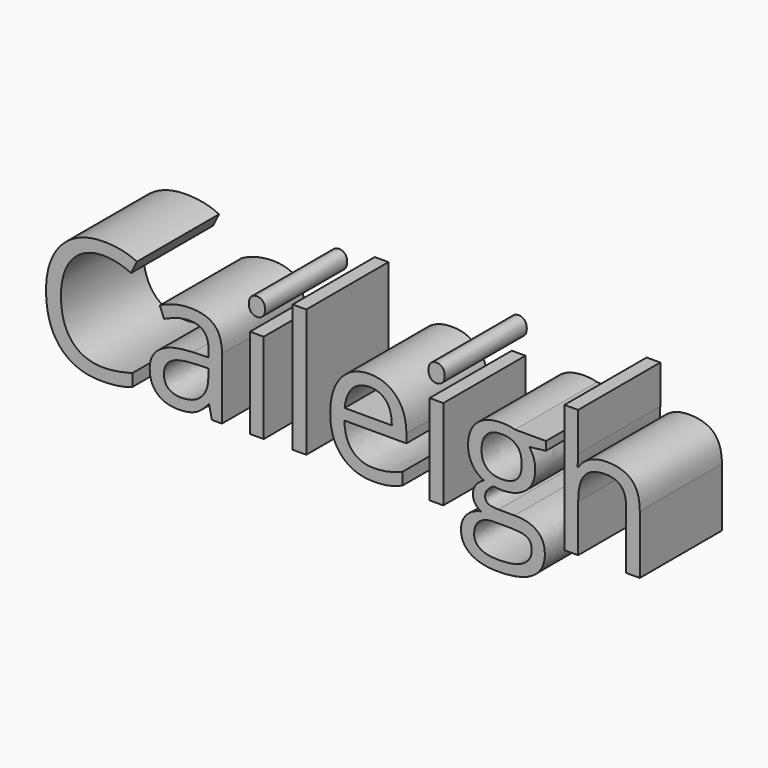
from build123d import *

# Parameters (mm, degrees)
F0_TEXT_SIZE = 41.6515395045
F1_DEPTH     = 25.4


# Not quite as in the source:
# - Text() gives the source's letters only with a copy of the font that has no kerning and outlines rounded to 1/6400 em; it was checked with that copy


with BuildPart() as f1:
    # F0 (on Front) → F1 (new body)
    with BuildSketch(Plane.XZ):
        with Locations((-72.8641599417, 21.4375257492)):
            Text('Caileigh', F0_TEXT_SIZE, font='Open Sans', text_align=(TextAlign.LEFT, TextAlign.BOTTOM))
    extrude(amount=F1_DEPTH)


solid = f1.part
